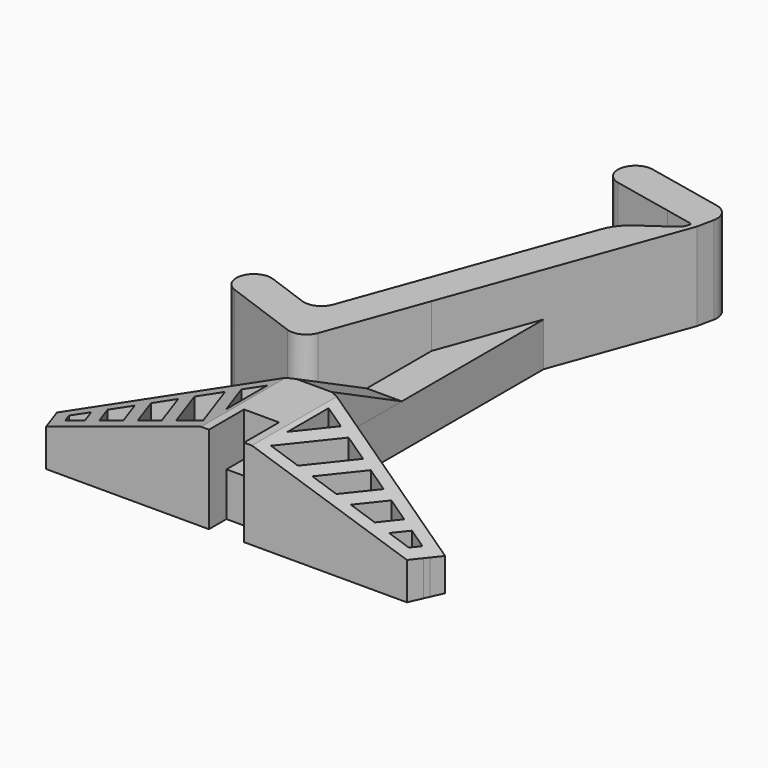
from build123d import *

# Parameters (mm, degrees)
F1_DEPTH     = 20
F0_W         = 4
F0_H         = 15
F2_TEXT_SIZE = 5.5555555556
F3_DEPTH     = 1
F4_R         = 3.99999
F5_R         = 10
F6_R         = 0.5
F7_R         = 3
F8_T1_DEPTH  = 40
F8_T3_DEPTH  = 39.9362007482
F9_DEPTH     = 10
F10_T1_DEPTH = 206.6870041307
F11_T1_DEPTH = 206.6870041307
F12_DEPTH    = 10
F14_DEPTH    = 8


# Not quite as in the source:
# - a fillet or chamfer that OpenCascade refuses, or shapes differently, is made with other operations: its cross-section is extruded or revolved along the edge and cut away or added
# - a fillet or chamfer is up to 0.001 mm smaller than in the source, because OpenCascade refuses the exact size
# - Text() gives the source's letters only with a copy of the font that has no kerning and outlines rounded to 1/6400 em; it was checked with that copy


with BuildPart() as f1:
    # F0 (on Top) → F1 (new body)
    with BuildSketch(Plane.XY):
        Polygon((4.4764376284, 52.2883313939), (-17.1019733182, -6.9978654297), (-34.0164404924, -0.8415028498), (-36.752601639, -8.3590438161), (-12.3205934985, -17.2515675426), (-2.8543493245, 8.7567245727), (5.1456506755, 30.7365439283), (16.0670783975, 60.7429199827), (17.686454988, 68.4830078278), (-7.7453826311, 73.888711789), (-9.4086761576, 66.0635309832), (8.1330941444, 62.3349126022), (14.8004769606, 60.9177166354), (14.1164366739, 59.0383313939), align=None)
    extrude(amount=F1_DEPTH)

    # F2 (on face) → F3 (cut)
    with BuildSketch(Plane(origin=(14.6918115418, 69.1195389422, 0), x_dir=(-0.9781476007, 0.2079116908, 0), z_dir=(0.2079116908, 0.9781476007, 0))):
        with Locations(Location((23.0249170735, 7.3618779402), (0, 0, 180))):
            Text('10 deg.', F2_TEXT_SIZE, font='Open Sans', font_style=FontStyle.BOLD, text_align=(TextAlign.LEFT, TextAlign.BOTTOM))
        with Locations(Location((23.0249170735, 14.9174334958), (0, 0, 180))):
            Text('1.25 mm', F2_TEXT_SIZE, font='Open Sans', font_style=FontStyle.BOLD, text_align=(TextAlign.LEFT, TextAlign.BOTTOM))
    extrude(amount=-F3_DEPTH, mode=Mode.SUBTRACT)

    # F4 (radius 4 in the source; OpenCascade refuses exactly that, so slightly less here)
    f4_edges = [f1.edges().sort_by_distance(p)[0] for p in [
        (-34.01644, -0.841503, 10),
        (-36.752602, -8.359044, 10),
        (-17.101973, -6.997865, 10),
        (-12.320593, -17.251568, 10),
    ]]
    fillet(f4_edges, radius=F4_R)

    # F5
    f5_edges = [f1.edges().sort_by_distance(p)[0] for p in [
        (4.476438, 52.288331, 10),
    ]]
    fillet(f5_edges, radius=F5_R)

    # F6
    f6_edges = [f1.edges().sort_by_distance(p)[0] for p in [
        (14.800477, 60.917717, 10),
    ]]
    fillet(f6_edges, radius=F6_R)

    # F7
    f7_edges = [f1.edges().sort_by_distance(p)[0] for p in [
        (14.116437, 59.038331, 10),
    ]]
    fillet(f7_edges, radius=F7_R)

    # F8: fillet of radius 4 on 3 edges, made by hand

    # F8_s2 → F8_t1 (cut)
    with BuildSketch(Plane.XY.offset(-10)):
        with BuildLine():
            ThreePointArc((-5.4960857547, 65.2318842199), (-8.0191212632, 66.9659184828), (-8.5770293943, 69.9761213861))
            Line((-8.5770293943, 69.9761213861), (-9.4086761576, 66.0635309832))
            Line((-9.4086761576, 66.0635309832), (-5.4960857547, 65.2318842199))
        make_face()
        with BuildLine():
            ThreePointArc((-8.5770293943, 69.9761213861), (-6.8429951315, 72.4991568946), (-3.8327922281, 73.0570650258))
            Line((-3.8327922281, 73.0570650258), (-7.7453826311, 73.888711789))
            Line((-7.7453826311, 73.888711789), (-8.5770293943, 69.9761213861))
        make_face()
    extrude(amount=F8_T1_DEPTH, mode=Mode.SUBTRACT)

    # F8_s4 → F8_t3 (cut)
    with BuildSketch(Plane.XY.offset(-9.9681003741)):
        with BuildLine():
            ThreePointArc((13.7863456021, 69.312001669), (16.305896527, 67.5833238226), (16.8699264246, 64.5802696716))
            Line((16.8699264246, 64.5802696716), (17.686454988, 68.4830078278))
            Line((17.686454988, 68.4830078278), (13.7863456021, 69.312001669))
        make_face()
    extrude(amount=F8_T3_DEPTH, mode=Mode.SUBTRACT)


with BuildPart() as f1b:
    # F0 (on Top) → F1, piece 2 (new body)
    with BuildSketch(Plane.XY):
        with Locations((-0.8543493245, -37.2515675426)):
            Rectangle(F0_W, F0_H)
        with Locations((3.1456506755, -37.2515675426)):
            Rectangle(F0_W, F0_H)
        Polygon((-2.8543493245, -44.7515675426), (-2.8543493245, -29.7515675426), (-43.1458000904, -47.7515675426), (-41.9221251536, -50.4906585686), (-39.1830341275, -49.2669836318), (-35.4367063239, -47.5933308052), (-32.6976152979, -46.3696558684), (-28.1324635877, -44.3301976404), (-25.3933725617, -43.1065227036), (-20.8282208516, -41.0670644756), (-18.0891298255, -39.8433895388), (-12.9527377755, -37.5487326044), (-10.2136467495, -36.3250576676), (-5.8543493245, -34.3775637909), (-5.8543493245, -46.0829697549), (-5.8543493245, -51.7515675426), (-6.6076937518, -51.7515675426), (-12.7692120764, -51.7515675426), (-16.0549736354, -51.7515675426), (-21.5312429003, -51.7515675426), (-24.8170044593, -51.7515675426), (-30.2932737243, -51.7515675426), (-33.5790352833, -51.7515675426), (-38.0730589456, -51.7515675426), (-41.3588205046, -51.7515675426), (-40.0185858153, -54.7515675426), (-2.8543493245, -54.7515675426), (-2.8543493245, -49.7515675426), align=None)
        Polygon((-10.2136467495, -36.3250576676), (-12.9527377755, -37.5487326044), (-6.6076937518, -51.7515675426), (-5.8543493245, -51.7515675426), (-5.8543493245, -46.0829697549), align=None)
        Polygon((-18.0891298255, -39.8433895388), (-20.8282208516, -41.0670644756), (-16.0549736354, -51.7515675426), (-12.7692120764, -51.7515675426), align=None)
        Polygon((-25.3933725617, -43.1065227036), (-28.1324635877, -44.3301976404), (-24.8170044593, -51.7515675426), (-21.5312429003, -51.7515675426), align=None)
        Polygon((-32.6976152979, -46.3696558684), (-35.4367063239, -47.5933308052), (-33.5790352833, -51.7515675426), (-30.2932737243, -51.7515675426), align=None)
        Polygon((-39.1830341275, -49.2669836318), (-41.9221251536, -50.4906585686), (-41.3588205046, -51.7515675426), (-38.0730589456, -51.7515675426), align=None)
        Polygon((-40.0185858153, -54.7515675426), (-41.3588205046, -51.7515675426), (-43.1458000904, -51.7515675426), (-43.1458000904, -54.7515675426), align=None)
        Polygon((-41.3588205046, -51.7515675426), (-41.9221251536, -50.4906585686), (-43.1458000904, -51.0373291015), (-43.1458000904, -51.7515675426), align=None)
        Polygon((-41.9221251536, -50.4906585686), (-43.1458000904, -47.7515675426), (-43.1458000904, -51.0373291015), align=None)
        Polygon((45.4371014414, -51.7515675426), (43.6501218557, -51.7515675426), (42.3098871663, -54.7515675426), (45.4371014414, -54.7515675426), align=None)
        Polygon((45.4371014414, -51.0373291015), (44.2134265046, -50.4906585686), (43.6501218557, -51.7515675426), (45.4371014414, -51.7515675426), align=None)
        Polygon((45.4371014414, -51.0373291015), (45.4371014414, -47.7515675426), (44.2134265046, -50.4906585686), align=None)
        Polygon((45.4371014414, -47.7515675426), (5.1456506755, -29.7515675426), (5.1456506755, -44.7515675426), (5.1456506755, -49.7515675426), (5.1456506755, -54.7515675426), (42.3098871663, -54.7515675426), (43.6501218557, -51.7515675426), (40.3643602967, -51.7515675426), (35.8703366343, -51.7515675426), (32.5845750753, -51.7515675426), (27.1083058104, -51.7515675426), (23.8225442514, -51.7515675426), (18.3462749864, -51.7515675426), (15.0605134274, -51.7515675426), (8.8989951029, -51.7515675426), (8.1456506755, -51.7515675426), (8.1456506755, -46.0829697549), (8.1456506755, -34.3775637909), (12.5049481005, -36.3250576676), (15.2440391266, -37.5487326044), (20.3804311766, -39.8433895388), (23.1195222026, -41.0670644756), (27.6846739127, -43.1065227036), (30.4237649388, -44.3301976404), (34.9889166489, -46.3696558684), (37.728007675, -47.5933308052), (41.4743354786, -49.2669836318), (44.2134265046, -50.4906585686), align=None)
        Polygon((43.6501218557, -51.7515675426), (44.2134265046, -50.4906585686), (41.4743354786, -49.2669836318), (40.3643602967, -51.7515675426), align=None)
        Polygon((35.8703366343, -51.7515675426), (37.728007675, -47.5933308052), (34.9889166489, -46.3696558684), (32.5845750753, -51.7515675426), align=None)
        Polygon((27.1083058104, -51.7515675426), (30.4237649388, -44.3301976404), (27.6846739127, -43.1065227036), (23.8225442514, -51.7515675426), align=None)
        Polygon((18.3462749864, -51.7515675426), (23.1195222026, -41.0670644756), (20.3804311766, -39.8433895388), (15.0605134274, -51.7515675426), align=None)
        Polygon((8.8989951029, -51.7515675426), (15.2440391266, -37.5487326044), (12.5049481005, -36.3250576676), (8.1456506755, -46.0829697549), (8.1456506755, -51.7515675426), align=None)
    extrude(amount=F1_DEPTH)

    # F10: chamfer of 12.5 x 38.4710442147 on 1 edges, made by hand

    # F10_s2 → F10_t1 (cut)
    with BuildSketch(Plane.XZ.offset(-52.0919345228)):
        Polygon((-43.1458000904, 7.5), (-4.6747558757, 20), (-43.1458000904, 20), align=None)
    extrude(amount=F10_T1_DEPTH, mode=Mode.SUBTRACT)

    # F11: chamfer of 12.5 x 38.4710442147 on 1 edges, made by hand

    # F11_s2 → F11_t1 (cut)
    with BuildSketch(Plane.XZ.offset(-52.0919345228)):
        Polygon((6.9660572267, 20), (45.4371014414, 7.5), (45.4371014414, 20), align=None)
    extrude(amount=F11_T1_DEPTH, mode=Mode.SUBTRACT)

    # F0 (on Top) → F12 (cut)
    with BuildSketch(Plane.XY):
        Polygon((-41.9221251536, -50.4906585686), (-43.1458000904, -47.7515675426), (-43.1458000904, -51.0373291015), align=None)
        Polygon((-41.3588205046, -51.7515675426), (-41.9221251536, -50.4906585686), (-43.1458000904, -51.0373291015), (-43.1458000904, -51.7515675426), align=None)
        Polygon((-40.0185858153, -54.7515675426), (-41.3588205046, -51.7515675426), (-43.1458000904, -51.7515675426), (-43.1458000904, -54.7515675426), align=None)
        Polygon((45.4371014414, -51.7515675426), (43.6501218557, -51.7515675426), (42.3098871663, -54.7515675426), (45.4371014414, -54.7515675426), align=None)
        Polygon((45.4371014414, -51.0373291015), (44.2134265046, -50.4906585686), (43.6501218557, -51.7515675426), (45.4371014414, -51.7515675426), align=None)
        Polygon((45.4371014414, -51.0373291015), (45.4371014414, -47.7515675426), (44.2134265046, -50.4906585686), align=None)
    extrude(amount=F12_DEPTH, mode=Mode.SUBTRACT)


with BuildPart() as f9:
    # F0 (on Top) → F9 (new body)
    with BuildSketch(Plane.XY):
        Polygon((5.1456506755, 30.7365439283), (-2.8543493245, 8.7567245727), (-2.8543493245, -29.7515675426), (1.1456506755, -29.7515675426), (5.1456506755, -29.7515675426), align=None)
    extrude(amount=F9_DEPTH)


with BuildPart() as f9b:
    # F0 (on Top) → F9, piece 2 (new body)
    with BuildSketch(Plane.XY):
        Polygon((1.1456506755, -44.7515675426), (-2.8543493245, -44.7515675426), (-2.8543493245, -49.7515675426), (5.1456506755, -49.7515675426), (5.1456506755, -44.7515675426), align=None)
    extrude(amount=F9_DEPTH)


with BuildPart() as f14:
    # F13 (on face) → F14 (new body)
    with BuildSketch(Plane.YZ.offset(5.1456506755)):
        Polygon((-29.7515675426, 20), (-29.7515675426, 10), (-9.7515675426, 10), align=None)
    extrude(amount=-F14_DEPTH)


solid = Compound([f1.part, f1b.part, f9.part, f9b.part, f14.part])
